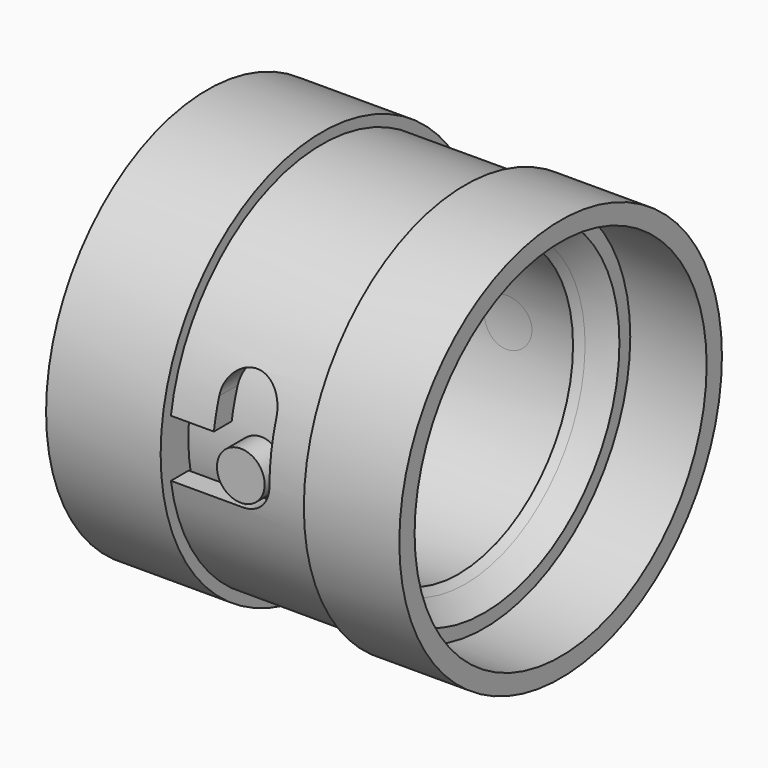
from build123d import *

# Parameters (mm, degrees)
F0_R           = 26.8224
F0_R_2         = 24.2824
F0_R_3         = 19.05
F1_DEPTH       = 2.54
F2_DEPTH       = 12.7
F3_R           = 25.4
F3_R_2         = 22.479
F4_DEPTH       = 19.05
F5_W           = 9.525
F5_H           = 7.62
F6_DEPTH       = 50.8
F6_DEPTH_BACK  = 50.8
F7_R           = 3.81
F8_DEPTH       = 50.8
F8_DEPTH_BACK  = 50.8
F10_DEPTH      = 50.8
F12_DEPTH      = 25.4
F13_R          = 22.225
F13_R_2        = 19.05
F14_DEPTH      = 21.59
F15_START      = -19.05
F13_R_3        = 24.2824
F15_DEPTH      = 2.54
F17_START      = -19.05
F16_R          = 26.8224
F16_R_2        = 24.2824
F17_DEPTH      = 15.24
F18_R          = 3.175
F19_DEPTH      = 25.4
F19_DEPTH_BACK = 25.4
F20_DEPTH      = 25.4
F21_W          = 2.54
F21_H          = 0.889


with BuildPart() as f1:
    # F0 (on Right) → F1 (new body)
    with BuildSketch(Plane.YZ):
        Circle(F0_R)
        Circle(F0_R_2, mode=Mode.SUBTRACT)
        Circle(F0_R_2)
        Circle(F0_R_3, mode=Mode.SUBTRACT)
    extrude(amount=F1_DEPTH)

    # F0 (on Right) → F2 (join)
    with BuildSketch(Plane.YZ):
        Circle(F0_R)
        Circle(F0_R_2, mode=Mode.SUBTRACT)
    extrude(amount=F2_DEPTH)

    # F3 (on Right) → F4 (join)
    with BuildSketch(Plane.YZ):
        Circle(F3_R)
        Circle(F3_R_2, mode=Mode.SUBTRACT)
    extrude(amount=-F4_DEPTH)

    # F5 (on Front) → F6 (cut, two sides)
    with BuildSketch(Plane.XZ) as f6_sk:
        with Locations((-14.2875, 0)):
            Rectangle(F5_W, F5_H)
    extrude(amount=-F6_DEPTH, mode=Mode.SUBTRACT)
    extrude(f6_sk.sketch, amount=F6_DEPTH_BACK, mode=Mode.SUBTRACT)

    # F7 (on Front) → F8 (cut, two sides)
    with BuildSketch(Plane.XZ) as f8_sk:
        with Locations((-9.525, 0)):
            Circle(F7_R)
    extrude(amount=-F8_DEPTH, mode=Mode.SUBTRACT)
    extrude(f8_sk.sketch, amount=F8_DEPTH_BACK, mode=Mode.SUBTRACT)

    # F9 (on Front) → F10 (cut)
    with BuildSketch(Plane.XZ):
        with BuildLine():
            ThreePointArc((-13.335, 7.62), (-9.525, 3.81), (-5.715, 7.62))
            ThreePointArc((-5.715, 7.62), (-9.525, 11.43), (-13.335, 7.62))
        make_face()
        with BuildLine():
            Line((-5.715, 0), (-5.715, 7.62))
            ThreePointArc((-5.715, 7.62), (-9.525, 3.81), (-13.335, 7.62))
            Line((-13.335, 7.62), (-13.335, 0))
            Line((-13.335, 0), (-5.715, 0))
        make_face()
    extrude(amount=F10_DEPTH, mode=Mode.SUBTRACT)

    # F11 (on Front) → F12 (cut)
    with BuildSketch(Plane.XZ):
        with BuildLine():
            ThreePointArc((-13.335, -7.62), (-9.525, -3.81), (-5.715, -7.62))
            Line((-5.715, -7.62), (-5.715, 0))
            Line((-5.715, 0), (-13.335, 0))
            Line((-13.335, 0), (-13.335, -7.62))
        make_face()
        with BuildLine():
            ThreePointArc((-13.335, -7.62), (-9.525, -11.43), (-5.715, -7.62))
            ThreePointArc((-5.715, -7.62), (-9.525, -3.81), (-13.335, -7.62))
        make_face()
    extrude(amount=-F12_DEPTH, mode=Mode.SUBTRACT)


with BuildPart() as f14:
    # F13 (on Right) → F14 (new body)
    with BuildSketch(Plane.YZ):
        Circle(F13_R)
        Circle(F13_R_2, mode=Mode.SUBTRACT)
    extrude(amount=-F14_DEPTH)

    # F13 (on Right) → F15 (join)
    with BuildSketch(Plane.YZ.offset(F15_START)):
        Circle(F13_R_3)
        Circle(F13_R, mode=Mode.SUBTRACT)
    extrude(amount=-F15_DEPTH)

    # F16 (on Right) → F17 (join)
    with BuildSketch(Plane.YZ.offset(F17_START)):
        Circle(F16_R)
        Circle(F16_R_2, mode=Mode.SUBTRACT)
    extrude(amount=-F17_DEPTH)

    # F18 (on Front) → F19 (join, two sides)
    with BuildSketch(Plane.XZ) as f19_sk:
        with Locations((-9.525, 0)):
            Circle(F18_R)
    extrude(amount=F19_DEPTH)
    extrude(f19_sk.sketch, amount=-F19_DEPTH_BACK)

    # F13 (on Right) → F20 (cut)
    with BuildSketch(Plane.YZ):
        Circle(F13_R_2)
    extrude(amount=-F20_DEPTH, mode=Mode.SUBTRACT)


with BuildPart() as f22_tool:
    # F21 (on Front) → F22 (revolve)
    with BuildSketch(Plane.XZ):
        Polygon((0, -19.939), (2.54, -22.479), (2.54, -19.939), align=None)
        with Locations((1.27, -19.4945)):
            Rectangle(F21_W, F21_H)
        Polygon((-0.889, -19.05), (0, -19.939), (0, -19.05), align=None)
    revolve(axis=Axis((12.2344479781, 0, 0), (1, 0, 0)))


with BuildPart() as f1_1:
    add(f1.part)

    # F22: cut by f22_tool
    add(f22_tool.part, mode=Mode.SUBTRACT)

    # F21 (on Front) → F25 (revolve, cut)
    with BuildSketch(Plane.XZ):
        Polygon((0, -19.939), (2.54, -22.479), (2.54, -19.939), align=None)
        with Locations((1.27, -19.4945)):
            Rectangle(F21_W, F21_H)
        Polygon((-0.889, -19.05), (0, -19.939), (0, -19.05), align=None)
    revolve(axis=Axis((12.2344479781, 0, 0), (1, 0, 0)), mode=Mode.SUBTRACT)


with BuildPart() as f14_1:
    add(f14.part)

    # F22: cut by f22_tool
    add(f22_tool.part, mode=Mode.SUBTRACT)

    # F23 (on Front) → F24 (revolve, cut)
    with BuildSketch(Plane.XZ):
        Polygon((-18.161, -19.05), (-21.59, -19.05), (-21.59, -22.479), align=None)
    revolve(axis=Axis((-10.795, 0, 0), (-1, 0, 0)), mode=Mode.SUBTRACT)


solid = Compound([f1_1.part, f14_1.part])
